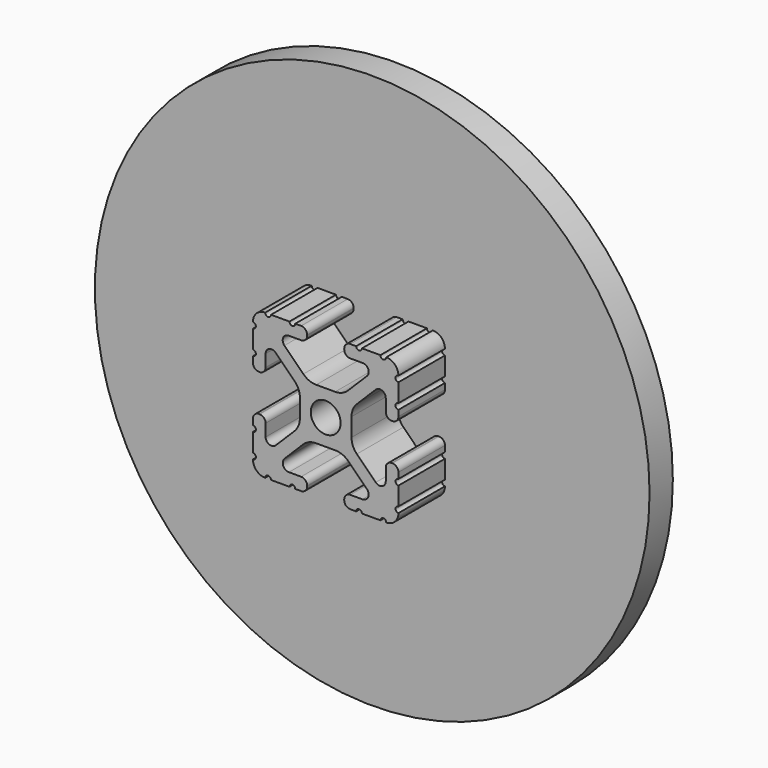
from build123d import *

# Parameters (mm, degrees)
F0_R     = 2.5625
F1_DEPTH = 12.5
F2_R     = 47.675
F2_R_2   = 17.675
F3_DEPTH = 2.5
F4_DEPTH = 12.5


# Not quite as in the source:
# - ends of sketch curves that miss each other by under 0.0002 mm in the source are joined
# - a feature of the source that left no trace in its solid (it failed there, or was rolled back) is left out


with BuildPart() as f1:
    # F0 (on Front) → F1 (new body, symmetric)
    with BuildSketch(Plane.XZ):
        with BuildLine():
            ThreePointArc((-3.8900202791, -5.3382797295), (-2.8768958758, -4.6623321828), (-1.682325, -4.425))
            Line((-1.682325, -4.425), (1.682325, -4.425))
            ThreePointArc((1.682325, -4.425), (2.8768958758, -4.6623321828), (3.8900202791, -5.3382797295))
            Line((3.8900202791, -5.3382797295), (7.066575, -8.50905))
            ThreePointArc((7.066575, -8.50905), (7.2979716135, -9.6681190856), (6.315375, -10.325))
            Line((6.315375, -10.325), (4.22, -10.325))
            ThreePointArc((4.22, -10.325), (3.4899122484, -10.6274122484), (3.1875, -11.3575))
            Line((3.1875, -11.3575), (3.1875, -11.4675))
            ThreePointArc((3.1875, -11.4675), (3.4899122484, -12.1975877516), (4.22, -12.5))
            Line((4.22, -12.5), (5.2334, -12.5))
            ThreePointArc((5.2334, -12.5), (5.7334, -12), (6.2334, -12.5))
            Line((6.2334, -12.5), (9.40005, -12.5))
            ThreePointArc((9.40005, -12.5), (9.899975, -12.0000000056), (10.4000499775, -12.49985))
            ThreePointArc((10.4000499775, -12.49985), (11.8922642472, -11.8922288945), (12.4998493922, -10.4000000073))
            ThreePointArc((12.4998493922, -10.4000000073), (12.0000000056, -9.899925), (12.5, -9.4))
            Line((12.5, -9.4), (12.5, -6.23335))
            ThreePointArc((12.5, -6.23335), (12, -5.73335), (12.5, -5.23335))
            Line((12.5, -5.23335), (12.5, -4.21995))
            ThreePointArc((12.5, -4.21995), (12.1975877516, -3.4898622484), (11.4675, -3.18745))
            Line((11.4675, -3.18745), (11.3575, -3.18745))
            ThreePointArc((11.3575, -3.18745), (10.6274122484, -3.4898622484), (10.325, -4.21995))
            Line((10.325, -4.21995), (10.325, -6.301275))
            ThreePointArc((10.325, -6.301275), (9.7012847872, -7.2353050667), (8.5995439137, -7.0171311001))
            Line((8.5995439137, -7.0171311001), (5.355325, -3.780325))
            ThreePointArc((5.355325, -3.780325), (4.6760601946, -2.7656350724), (4.4375, -1.5681))
            Line((4.4375, -1.5681), (4.4375, 1.5681))
            ThreePointArc((4.4375, 1.5681), (4.6760601946, 2.7656350724), (5.3553177597, 3.7803322568))
            Line((5.3553177597, 3.7803322568), (8.59955, 7.017125))
            ThreePointArc((8.59955, 7.017125), (9.7012847872, 7.2353050667), (10.325, 6.301275))
            Line((10.325, 6.301275), (10.325, 4.21995))
            ThreePointArc((10.325, 4.21995), (10.6274122484, 3.4898622484), (11.3575, 3.18745))
            Line((11.3575, 3.18745), (11.4675, 3.18745))
            ThreePointArc((11.4675, 3.18745), (12.1975877516, 3.4898622484), (12.5, 4.21995))
            Line((12.5, 4.21995), (12.5, 5.23335))
            ThreePointArc((12.5, 5.23335), (12, 5.73335), (12.5, 6.23335))
            Line((12.5, 6.23335), (12.5, 9.4))
            ThreePointArc((12.5, 9.4), (12.0000000056, 9.899925), (12.49985, 10.3999999775))
            ThreePointArc((12.49985, 10.3999999775), (11.8922642472, 11.8922288945), (10.40005, 12.499849994))
            ThreePointArc((10.40005, 12.499849994), (9.899975, 12.0000000056), (9.40005, 12.5))
            Line((9.40005, 12.5), (6.2334, 12.5))
            ThreePointArc((6.2334, 12.5), (5.7334, 12), (5.2334, 12.5))
            Line((5.2334, 12.5), (4.22, 12.5))
            ThreePointArc((4.22, 12.5), (3.4899122484, 12.1975877516), (3.1875, 11.4675))
            Line((3.1875, 11.4675), (3.1875, 11.3575))
            ThreePointArc((3.1875, 11.3575), (3.4899122484, 10.6274122484), (4.22, 10.325))
            Line((4.22, 10.325), (6.3748, 10.325))
            ThreePointArc((6.3748, 10.325), (7.3151859964, 9.696264211), (7.0935440721, 8.5869809415))
            Line((7.0935440721, 8.5869809415), (3.836875, 5.337775))
            ThreePointArc((3.836875, 5.337775), (2.8239359895, 4.6621936697), (1.6297, 4.425))
            Line((1.6297, 4.425), (-1.6297, 4.425))
            ThreePointArc((-1.6297, 4.425), (-2.8239359895, 4.6621936697), (-3.8368822403, 5.3377677432))
            Line((-3.8368822403, 5.3377677432), (-7.09355, 8.586975))
            ThreePointArc((-7.09355, 8.586975), (-7.3151859964, 9.696264211), (-6.3748, 10.325))
            Line((-6.3748, 10.325), (-4.22, 10.325))
            ThreePointArc((-4.22, 10.325), (-3.4899122484, 10.6274122484), (-3.1875, 11.3575))
            Line((-3.1875, 11.3575), (-3.1875, 11.4675))
            ThreePointArc((-3.1875, 11.4675), (-3.4899122484, 12.1975877516), (-4.22, 12.5))
            Line((-4.22, 12.5), (-5.2334, 12.5))
            ThreePointArc((-5.2334, 12.5), (-5.7334, 12), (-6.2334, 12.5))
            Line((-6.2334, 12.5), (-9.40005, 12.5))
            ThreePointArc((-9.40005, 12.5), (-9.899975, 12.0000000056), (-10.4000499775, 12.49985))
            ThreePointArc((-10.4000499775, 12.49985), (-11.8922642472, 11.8922288945), (-12.4998493922, 10.4000000073))
            ThreePointArc((-12.4998493922, 10.4000000073), (-12.0000000056, 9.899925), (-12.5, 9.4))
            Line((-12.5, 9.4), (-12.5, 6.23335))
            ThreePointArc((-12.5, 6.23335), (-12, 5.73335), (-12.5, 5.23335))
            Line((-12.5, 5.23335), (-12.5, 4.21995))
            ThreePointArc((-12.5, 4.21995), (-12.1975877516, 3.4898622484), (-11.4675, 3.18745))
            Line((-11.4675, 3.18745), (-11.3575, 3.18745))
            ThreePointArc((-11.3575, 3.18745), (-10.6274122484, 3.4898622484), (-10.325, 4.21995))
            Line((-10.325, 4.21995), (-10.325, 6.301275))
            ThreePointArc((-10.325, 6.301275), (-9.7012847872, 7.2353050667), (-8.5995439137, 7.0171311001))
            Line((-8.5995439137, 7.0171311001), (-5.355325, 3.780325))
            ThreePointArc((-5.355325, 3.780325), (-4.6760601946, 2.7656350724), (-4.4375, 1.5681))
            Line((-4.4375, 1.5681), (-4.4375, -1.5681))
            ThreePointArc((-4.4375, -1.5681), (-4.6760601946, -2.7656350724), (-5.3553177597, -3.7803322568))
            Line((-5.3553177597, -3.7803322568), (-8.59955, -7.017125))
            ThreePointArc((-8.59955, -7.017125), (-9.7012847872, -7.2353050667), (-10.325, -6.301275))
            Line((-10.325, -6.301275), (-10.325, -4.21995))
            ThreePointArc((-10.325, -4.21995), (-10.6274122484, -3.4898622484), (-11.3575, -3.18745))
            Line((-11.3575, -3.18745), (-11.4675, -3.18745))
            ThreePointArc((-11.4675, -3.18745), (-12.1975877516, -3.4898622484), (-12.5, -4.21995))
            Line((-12.5, -4.21995), (-12.5, -5.23335))
            ThreePointArc((-12.5, -5.23335), (-12, -5.73335), (-12.5, -6.23335))
            Line((-12.5, -6.23335), (-12.5, -9.4))
            ThreePointArc((-12.5, -9.4), (-12.0000000056, -9.899925), (-12.49985, -10.3999999775))
            ThreePointArc((-12.49985, -10.3999999775), (-11.8922642472, -11.8922288945), (-10.40005, -12.499849994))
            ThreePointArc((-10.40005, -12.499849994), (-9.899975, -12.0000000056), (-9.40005, -12.5))
            Line((-9.40005, -12.5), (-6.2334, -12.5))
            ThreePointArc((-6.2334, -12.5), (-5.7334, -12), (-5.2334, -12.5))
            Line((-5.2334, -12.5), (-4.22, -12.5))
            ThreePointArc((-4.22, -12.5), (-3.4899122484, -12.1975877516), (-3.1875, -11.4675))
            Line((-3.1875, -11.4675), (-3.1875, -11.3575))
            ThreePointArc((-3.1875, -11.3575), (-3.4899122484, -10.6274122484), (-4.22, -10.325))
            Line((-4.22, -10.325), (-6.315375, -10.325))
            ThreePointArc((-6.315375, -10.325), (-7.2979716135, -9.6681190856), (-7.0665766684, -8.5090483285))
            Line((-7.0665766684, -8.5090483285), (-3.8900202791, -5.3382797295))
        make_face()
        Circle(F0_R, mode=Mode.SUBTRACT)
    extrude(amount=F1_DEPTH, both=True)


with BuildPart() as f3:
    # F2 (on Front) → F3 (new body, symmetric)
    with BuildSketch(Plane.XZ):
        Circle(F2_R)
        Circle(F2_R_2, mode=Mode.SUBTRACT)
        Circle(F2_R_2)
    extrude(amount=F3_DEPTH, both=True)

    # F0 (on Front) → F4 (cut, symmetric)
    with BuildSketch(Plane.XZ):
        with BuildLine():
            ThreePointArc((-3.8900202791, -5.3382797295), (-2.8768958758, -4.6623321828), (-1.682325, -4.425))
            Line((-1.682325, -4.425), (1.682325, -4.425))
            ThreePointArc((1.682325, -4.425), (2.8768958758, -4.6623321828), (3.8900202791, -5.3382797295))
            Line((3.8900202791, -5.3382797295), (7.066575, -8.50905))
            ThreePointArc((7.066575, -8.50905), (7.2979716135, -9.6681190856), (6.315375, -10.325))
            Line((6.315375, -10.325), (4.22, -10.325))
            ThreePointArc((4.22, -10.325), (3.4899122484, -10.6274122484), (3.1875, -11.3575))
            Line((3.1875, -11.3575), (3.1875, -11.4675))
            ThreePointArc((3.1875, -11.4675), (3.4899122484, -12.1975877516), (4.22, -12.5))
            Line((4.22, -12.5), (5.2334, -12.5))
            ThreePointArc((5.2334, -12.5), (5.7334, -12), (6.2334, -12.5))
            Line((6.2334, -12.5), (9.40005, -12.5))
            ThreePointArc((9.40005, -12.5), (9.899975, -12.0000000056), (10.4000499775, -12.49985))
            ThreePointArc((10.4000499775, -12.49985), (11.8922642472, -11.8922288945), (12.4998493922, -10.4000000073))
            ThreePointArc((12.4998493922, -10.4000000073), (12.0000000056, -9.899925), (12.5, -9.4))
            Line((12.5, -9.4), (12.5, -6.23335))
            ThreePointArc((12.5, -6.23335), (12, -5.73335), (12.5, -5.23335))
            Line((12.5, -5.23335), (12.5, -4.21995))
            ThreePointArc((12.5, -4.21995), (12.1975877516, -3.4898622484), (11.4675, -3.18745))
            Line((11.4675, -3.18745), (11.3575, -3.18745))
            ThreePointArc((11.3575, -3.18745), (10.6274122484, -3.4898622484), (10.325, -4.21995))
            Line((10.325, -4.21995), (10.325, -6.301275))
            ThreePointArc((10.325, -6.301275), (9.7012847872, -7.2353050667), (8.5995439137, -7.0171311001))
            Line((8.5995439137, -7.0171311001), (5.355325, -3.780325))
            ThreePointArc((5.355325, -3.780325), (4.6760601946, -2.7656350724), (4.4375, -1.5681))
            Line((4.4375, -1.5681), (4.4375, 1.5681))
            ThreePointArc((4.4375, 1.5681), (4.6760601946, 2.7656350724), (5.3553177597, 3.7803322568))
            Line((5.3553177597, 3.7803322568), (8.59955, 7.017125))
            ThreePointArc((8.59955, 7.017125), (9.7012847872, 7.2353050667), (10.325, 6.301275))
            Line((10.325, 6.301275), (10.325, 4.21995))
            ThreePointArc((10.325, 4.21995), (10.6274122484, 3.4898622484), (11.3575, 3.18745))
            Line((11.3575, 3.18745), (11.4675, 3.18745))
            ThreePointArc((11.4675, 3.18745), (12.1975877516, 3.4898622484), (12.5, 4.21995))
            Line((12.5, 4.21995), (12.5, 5.23335))
            ThreePointArc((12.5, 5.23335), (12, 5.73335), (12.5, 6.23335))
            Line((12.5, 6.23335), (12.5, 9.4))
            ThreePointArc((12.5, 9.4), (12.0000000056, 9.899925), (12.49985, 10.3999999775))
            ThreePointArc((12.49985, 10.3999999775), (11.8922642472, 11.8922288945), (10.40005, 12.499849994))
            ThreePointArc((10.40005, 12.499849994), (9.899975, 12.0000000056), (9.40005, 12.5))
            Line((9.40005, 12.5), (6.2334, 12.5))
            ThreePointArc((6.2334, 12.5), (5.7334, 12), (5.2334, 12.5))
            Line((5.2334, 12.5), (4.22, 12.5))
            ThreePointArc((4.22, 12.5), (3.4899122484, 12.1975877516), (3.1875, 11.4675))
            Line((3.1875, 11.4675), (3.1875, 11.3575))
            ThreePointArc((3.1875, 11.3575), (3.4899122484, 10.6274122484), (4.22, 10.325))
            Line((4.22, 10.325), (6.3748, 10.325))
            ThreePointArc((6.3748, 10.325), (7.3151859964, 9.696264211), (7.0935440721, 8.5869809415))
            Line((7.0935440721, 8.5869809415), (3.836875, 5.337775))
            ThreePointArc((3.836875, 5.337775), (2.8239359895, 4.6621936697), (1.6297, 4.425))
            Line((1.6297, 4.425), (-1.6297, 4.425))
            ThreePointArc((-1.6297, 4.425), (-2.8239359895, 4.6621936697), (-3.8368822403, 5.3377677432))
            Line((-3.8368822403, 5.3377677432), (-7.09355, 8.586975))
            ThreePointArc((-7.09355, 8.586975), (-7.3151859964, 9.696264211), (-6.3748, 10.325))
            Line((-6.3748, 10.325), (-4.22, 10.325))
            ThreePointArc((-4.22, 10.325), (-3.4899122484, 10.6274122484), (-3.1875, 11.3575))
            Line((-3.1875, 11.3575), (-3.1875, 11.4675))
            ThreePointArc((-3.1875, 11.4675), (-3.4899122484, 12.1975877516), (-4.22, 12.5))
            Line((-4.22, 12.5), (-5.2334, 12.5))
            ThreePointArc((-5.2334, 12.5), (-5.7334, 12), (-6.2334, 12.5))
            Line((-6.2334, 12.5), (-9.40005, 12.5))
            ThreePointArc((-9.40005, 12.5), (-9.899975, 12.0000000056), (-10.4000499775, 12.49985))
            ThreePointArc((-10.4000499775, 12.49985), (-11.8922642472, 11.8922288945), (-12.4998493922, 10.4000000073))
            ThreePointArc((-12.4998493922, 10.4000000073), (-12.0000000056, 9.899925), (-12.5, 9.4))
            Line((-12.5, 9.4), (-12.5, 6.23335))
            ThreePointArc((-12.5, 6.23335), (-12, 5.73335), (-12.5, 5.23335))
            Line((-12.5, 5.23335), (-12.5, 4.21995))
            ThreePointArc((-12.5, 4.21995), (-12.1975877516, 3.4898622484), (-11.4675, 3.18745))
            Line((-11.4675, 3.18745), (-11.3575, 3.18745))
            ThreePointArc((-11.3575, 3.18745), (-10.6274122484, 3.4898622484), (-10.325, 4.21995))
            Line((-10.325, 4.21995), (-10.325, 6.301275))
            ThreePointArc((-10.325, 6.301275), (-9.7012847872, 7.2353050667), (-8.5995439137, 7.0171311001))
            Line((-8.5995439137, 7.0171311001), (-5.355325, 3.780325))
            ThreePointArc((-5.355325, 3.780325), (-4.6760601946, 2.7656350724), (-4.4375, 1.5681))
            Line((-4.4375, 1.5681), (-4.4375, -1.5681))
            ThreePointArc((-4.4375, -1.5681), (-4.6760601946, -2.7656350724), (-5.3553177597, -3.7803322568))
            Line((-5.3553177597, -3.7803322568), (-8.59955, -7.017125))
            ThreePointArc((-8.59955, -7.017125), (-9.7012847872, -7.2353050667), (-10.325, -6.301275))
            Line((-10.325, -6.301275), (-10.325, -4.21995))
            ThreePointArc((-10.325, -4.21995), (-10.6274122484, -3.4898622484), (-11.3575, -3.18745))
            Line((-11.3575, -3.18745), (-11.4675, -3.18745))
            ThreePointArc((-11.4675, -3.18745), (-12.1975877516, -3.4898622484), (-12.5, -4.21995))
            Line((-12.5, -4.21995), (-12.5, -5.23335))
            ThreePointArc((-12.5, -5.23335), (-12, -5.73335), (-12.5, -6.23335))
            Line((-12.5, -6.23335), (-12.5, -9.4))
            ThreePointArc((-12.5, -9.4), (-12.0000000056, -9.899925), (-12.49985, -10.3999999775))
            ThreePointArc((-12.49985, -10.3999999775), (-11.8922642472, -11.8922288945), (-10.40005, -12.499849994))
            ThreePointArc((-10.40005, -12.499849994), (-9.899975, -12.0000000056), (-9.40005, -12.5))
            Line((-9.40005, -12.5), (-6.2334, -12.5))
            ThreePointArc((-6.2334, -12.5), (-5.7334, -12), (-5.2334, -12.5))
            Line((-5.2334, -12.5), (-4.22, -12.5))
            ThreePointArc((-4.22, -12.5), (-3.4899122484, -12.1975877516), (-3.1875, -11.4675))
            Line((-3.1875, -11.4675), (-3.1875, -11.3575))
            ThreePointArc((-3.1875, -11.3575), (-3.4899122484, -10.6274122484), (-4.22, -10.325))
            Line((-4.22, -10.325), (-6.315375, -10.325))
            ThreePointArc((-6.315375, -10.325), (-7.2979716135, -9.6681190856), (-7.0665766684, -8.5090483285))
            Line((-7.0665766684, -8.5090483285), (-3.8900202791, -5.3382797295))
        make_face()
        Circle(F0_R, mode=Mode.SUBTRACT)
        Circle(F0_R)
    extrude(amount=F4_DEPTH, both=True, mode=Mode.SUBTRACT)


solid = Compound([f1.part, f3.part])
